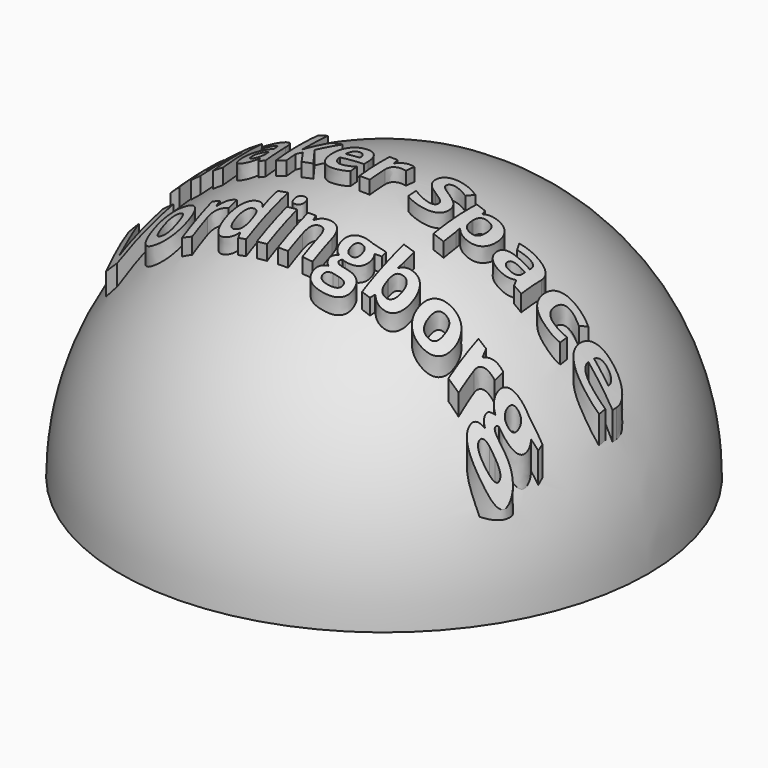
from build123d import *

# Parameters (mm, degrees)
F2_TEXT_SIZE = 7.8293208064
F4_DEPTH     = 25


# Not quite as in the source:
# - Text() gives the source's letters only with a copy of the font that has no kerning and outlines rounded to 1/6400 em; it was checked with that copy


with BuildPart() as f3:
    # F0 (on Front) → F3 (revolve)
    with BuildSketch(Plane.XZ):
        with BuildLine():
            Line((0, 0), (30, 0))
            ThreePointArc((30, 0), (21.2132034356, 21.2132034356), (0, 30))
            Line((0, 30), (0, 0))
        make_face()
    revolve(axis=Axis((0, 0, 15), (0, 0, 1)))

    # F2 (on offset) → F4 (join)
    with BuildSketch(Plane.XY.offset(35)):
        with Locations((-22.3990083252, -3.2549245619)):
            Text('Maker Space', F2_TEXT_SIZE, font='Open Sans', font_style=FontStyle.BOLD, text_align=(TextAlign.LEFT, TextAlign.BOTTOM))
        with Locations((-22.3990083252, -13.9028008586)):
            Text('Vordingborg', F2_TEXT_SIZE, font='Open Sans', font_style=FontStyle.BOLD, text_align=(TextAlign.LEFT, TextAlign.BOTTOM))
    extrude(amount=-F4_DEPTH)

    # F5 (on Front) → F6 (revolve, cut)
    with BuildSketch(Plane.XZ):
        with BuildLine():
            ThreePointArc((0, 31.5), (22.2738636074, 22.2738636074), (31.5, 0))
            Line((31.5, 0), (47.9393044887, 0))
            ThreePointArc((47.9393044887, 0), (33.8982072894, 33.8982072894), (0, 47.9393044887))
            Line((0, 47.9393044887), (0, 31.5))
        make_face()
    revolve(axis=Axis((0, 0, 39.7196522444), (0, 0, 1)), mode=Mode.SUBTRACT)


solid = f3.part
